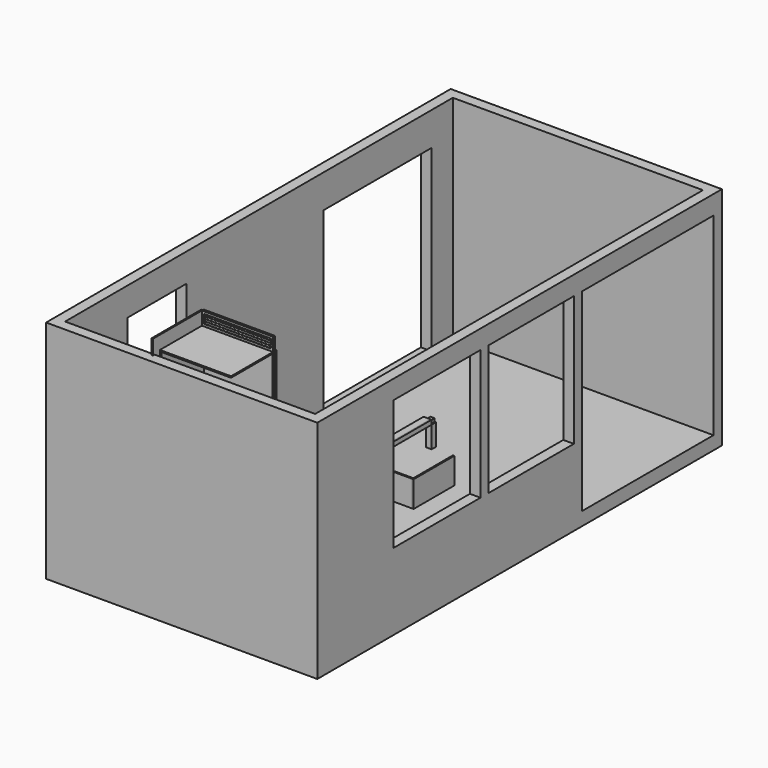
from build123d import *

# Parameters (mm, degrees)
F0_W      = 3098.8
F0_H      = 5778.5
F1_DEPTH  = 152.4
F2_W      = 3098.8
F2_H      = 5778.5
F2_W_2    = 2857.5
F2_H_2    = 5537.2
F3_DEPTH  = 2425.7
F4_W      = 1879.6
F4_H      = 2209.8
F5_DEPTH  = 120.65
F6_W      = 1219.2
F6_H      = 1485.9
F6_W_2    = 1244.6
F7_DEPTH  = 120.65
F8_W      = 844.55
F8_H      = 914.4
F9_DEPTH  = 120.651
F10_W     = 1543.05
F10_H     = 2044.7
F11_DEPTH = 120.651
F13_W     = 812.8
F13_H     = 609.6
F14_DEPTH = 15.875
F15_W     = 781.05
F15_H     = 476.25
F16_DEPTH = 15.875
F15_W_2   = 15.875
F17_DEPTH = 609.6
F18_DEPTH = 15.875
F19_W     = 812.8
F19_H     = 508
F19_W_2   = 781.05
F19_H_2   = 476.25
F19_W_3   = 711.2
F19_H_3   = 406.4
F20_DEPTH = 25.4
F21_W     = 4.7752
F21_H     = 12.7
F24_W     = 736.6
F24_H     = 431.8
F25_DEPTH = 4.7752
F29_W     = 812.8
F29_H     = 152.4
F29_W_2   = 762
F29_H_2   = 101.6
F30_DEPTH = 25.4
F32_DEPTH = 787.4
F34_DEPTH = 15.875
F35_W     = 76.2
F35_H     = 15.875
F36_DEPTH = 984.25
F38_DEPTH = 984.25
F39_W     = 15.875
F39_H     = 50.8
F40_DEPTH = 984.25
F42_DEPTH = 63.5
F43_W     = 565.15
F43_H     = 15.875
F44_DEPTH = 15.875
F45_W     = 609.6
F45_H     = 476.25
F46_DEPTH = 15.875


with BuildPart() as f1:
    # F0 (on Top) → F1 (new body)
    with BuildSketch(Plane.XY):
        Rectangle(F0_W, F0_H)
    extrude(amount=F1_DEPTH)

    # F2 (on face) → F3 (join)
    with BuildSketch(Plane.XY.offset(152.4)):
        Rectangle(F2_W, F2_H)
        Rectangle(F2_W_2, F2_H_2, mode=Mode.SUBTRACT)
    extrude(amount=F3_DEPTH)

    # F4 (on face) → F5 (cut, through all)
    with BuildSketch(Plane.YZ.offset(1549.4)):
        with Locations((1828.8, 1257.3)):
            Rectangle(F4_W, F4_H)
    extrude(amount=-F5_DEPTH, mode=Mode.SUBTRACT)

    # F6 (on face) → F7 (cut, through all)
    with BuildSketch(Plane.YZ.offset(1549.4)):
        with Locations((165.1, 1619.25)):
            Rectangle(F6_W, F6_H)
        with Locations((-1181.1, 1619.25)):
            Rectangle(F6_W_2, F6_H)
    extrude(amount=-F7_DEPTH, mode=Mode.SUBTRACT)

    # F8 (on face) → F9 (cut, through all)
    with BuildSketch(Plane.YZ.offset(-1428.75)):
        with Locations((-1457.325, 1797.05)):
            Rectangle(F8_W, F8_H)
    extrude(amount=-F9_DEPTH, mode=Mode.SUBTRACT)

    # F10 (on face) → F11 (cut, through all)
    with BuildSketch(Plane.YZ.offset(-1428.75)):
        with Locations((1692.275, 1174.75)):
            Rectangle(F10_W, F10_H)
    extrude(amount=-F11_DEPTH, mode=Mode.SUBTRACT)


with BuildPart() as f14:
    # F13 (on face) → F14 (new body)
    with BuildSketch(Plane.XY.offset(2578.1)):
        with Locations((0, -2387.6)):
            Rectangle(F13_W, F13_H)
    extrude(amount=F14_DEPTH)


with BuildPart() as f16:
    # F15 (on face) → F16 (new body)
    with BuildSketch(Plane(origin=(0, -2082.8, 0), x_dir=(-1, 0, 0), z_dir=(0, 1, 0))):
        with Locations((0, 2339.975)):
            Rectangle(F15_W, F15_H)
    extrude(amount=F16_DEPTH)


with BuildPart() as f17:
    # F15 (on face) → F17 (new body, through all)
    with BuildSketch(Plane(origin=(0, -2082.8, 0), x_dir=(-1, 0, 0), z_dir=(0, 1, 0))):
        with Locations((398.4625, 2339.975)):
            Rectangle(F15_W_2, F15_H)
    extrude(amount=-F17_DEPTH)


with BuildPart() as f18:
    # F15 (on face) → F18 (new body)
    with BuildSketch(Plane(origin=(0, -2082.8, 0), x_dir=(-1, 0, 0), z_dir=(0, 1, 0))):
        with Locations((0, 2339.975)):
            Rectangle(F15_W, F15_H)
    extrude(amount=F18_DEPTH)


with BuildPart() as f20:
    # F19 (on face) → F20 (new body)
    with BuildSketch(Plane(origin=(0, -2066.925, 0), x_dir=(-1, 0, 0), z_dir=(0, 1, 0))):
        with Locations((0, 2339.975)):
            Rectangle(F19_W, F19_H)
        with Locations((0, 2339.975)):
            Rectangle(F19_W_2, F19_H_2, mode=Mode.SUBTRACT)
        with Locations((0, 2339.975)):
            Rectangle(F19_W_2, F19_H_2)
        with Locations((0, 2339.975)):
            Rectangle(F19_W_3, F19_H_3, mode=Mode.SUBTRACT)
    extrude(amount=F20_DEPTH)

    # F23: sweep along a path in F22
    with BuildLine(Plane(origin=(0, -2041.525, 0), x_dir=(-1, 0, 0), z_dir=(0, 1, 0))) as f23_path:
        Line((355.6, 2543.175), (-355.6, 2543.175))
        Line((-355.6, 2543.175), (-355.6, 2136.775))
        Line((-355.6, 2136.775), (355.6, 2136.775))
        Line((355.6, 2136.775), (355.6, 2543.175))
    # F21 (on face) → F23 (sweep, cut)
    with BuildSketch(Plane(origin=(355.6, 0, 0), x_dir=(0, -1, 0), z_dir=(-1, 0, 0))):
        with Locations((2043.9126, 2130.425)):
            Rectangle(F21_W, F21_H)
    sweep(path=f23_path.line, transition=Transition.RIGHT, mode=Mode.SUBTRACT)


with BuildPart() as f25:
    # F24 (on face) → F25 (new body)
    with BuildSketch(Plane(origin=(0, -2041.525, 0), x_dir=(-1, 0, 0), z_dir=(0, 1, 0))):
        with Locations((0, 2339.975)):
            Rectangle(F24_W, F24_H)
    extrude(amount=F25_DEPTH)


with BuildPart() as f28:
    # F28: sweep along a path in F26
    with BuildLine(Plane(origin=(0, 0, 2085.975), x_dir=(1, 0, 0), z_dir=(0, 0, -1))) as f28_path:
        Line((63.5, 2066.925), (63.5, 2092.325))
        ThreePointArc((63.5, 2092.325), (59.7802561211, 2101.3052561211), (50.8, 2105.025))
        Line((50.8, 2105.025), (-50.8, 2105.025))
        ThreePointArc((-50.8, 2105.025), (-59.7802561211, 2101.3052561211), (-63.5, 2092.325))
        Line((-63.5, 2092.325), (-63.5, 2066.925))
    # F27 (on face) → F28 (sweep)
    with BuildSketch(Plane.XZ.offset(2066.925)):
        with BuildLine():
            ThreePointArc((57.15, 2085.975), (63.5, 2079.625), (69.85, 2085.975))
            Line((69.85, 2085.975), (57.15, 2085.975))
        make_face()
        with BuildLine():
            Line((57.15, 2085.975), (69.85, 2085.975))
            ThreePointArc((69.85, 2085.975), (63.5, 2092.325), (57.15, 2085.975))
        make_face()
    sweep(path=f28_path.line)


with BuildPart() as f30:
    # F29 (on face) → F30 (new body)
    with BuildSketch(Plane.XZ.offset(2066.925)):
        with Locations((0, 2670.175)):
            Rectangle(F29_W, F29_H)
        with Locations((0, 2670.175)):
            Rectangle(F29_W_2, F29_H_2, mode=Mode.SUBTRACT)
    extrude(amount=F30_DEPTH)

    # F31 (on face) → F32 (join, through all)
    with BuildSketch(Plane(origin=(-406.4, 0, 0), x_dir=(0, -1, 0), z_dir=(-1, 0, 0))):
        with BuildLine():
            Line((2068.3996798487, 2715.0101920908), (2086.3601920908, 2697.0496798487))
            ThreePointArc((2086.3601920908, 2697.0496798487), (2090.8503201513, 2697.0496798487), (2090.8503201513, 2701.5398079092))
            Line((2090.8503201513, 2701.5398079092), (2072.8898079092, 2719.5003201513))
            ThreePointArc((2072.8898079092, 2719.5003201513), (2068.3996798487, 2719.5003201513), (2068.3996798487, 2715.0101920908))
        make_face()
        with BuildLine():
            Line((2068.3996798487, 2689.6101920908), (2086.3601920908, 2671.6496798487))
            ThreePointArc((2086.3601920908, 2671.6496798487), (2090.8503201513, 2671.6496798487), (2090.8503201513, 2676.1398079092))
            Line((2090.8503201513, 2676.1398079092), (2072.8898079092, 2694.1003201513))
            ThreePointArc((2072.8898079092, 2694.1003201513), (2068.3996798487, 2694.1003201513), (2068.3996798487, 2689.6101920908))
        make_face()
        with BuildLine():
            Line((2068.3996798487, 2664.2101920908), (2086.3601920908, 2646.2496798487))
            ThreePointArc((2086.3601920908, 2646.2496798487), (2090.8503201513, 2646.2496798487), (2090.8503201513, 2650.7398079092))
            Line((2090.8503201513, 2650.7398079092), (2072.8898079092, 2668.7003201513))
            ThreePointArc((2072.8898079092, 2668.7003201513), (2068.3996798487, 2668.7003201513), (2068.3996798487, 2664.2101920908))
        make_face()
        with BuildLine():
            Line((2090.8503201513, 2625.3398079092), (2072.8898079092, 2643.3003201513))
            ThreePointArc((2072.8898079092, 2643.3003201513), (2068.3996798487, 2643.3003201513), (2068.3996798487, 2638.8101920908))
            Line((2068.3996798487, 2638.8101920908), (2086.3601920908, 2620.8496798487))
            ThreePointArc((2086.3601920908, 2620.8496798487), (2090.8503201513, 2620.8496798487), (2090.8503201513, 2625.3398079092))
        make_face()
    extrude(amount=-F32_DEPTH)


with BuildPart() as f34:
    # F33 (on Front) → F34 (new body)
    with BuildSketch(Plane.XZ):
        Polygon((335.1245088988, 450.85), (-335.1245088988, 450.85), (-335.1245088988, -450.85), (258.9245088988, -450.85), (258.9245088988, -323.85), (335.1245088988, -323.85), align=None)
    extrude(amount=F34_DEPTH)


with BuildPart() as f36:
    # F35 (on face) → F36 (new body)
    with BuildSketch(Plane(origin=(0, 0, 0), x_dir=(-1, 0, 0), z_dir=(0, 1, 0))):
        with Locations((297.0245088988, 442.9125)):
            Rectangle(F35_W, F35_H)
    extrude(amount=F36_DEPTH)


with BuildPart() as f38:
    # F37 (on face) → F38 (new body)
    with BuildSketch(Plane(origin=(0, 0, 0), x_dir=(-1, 0, 0), z_dir=(0, 1, 0))):
        Polygon((335.1245088988, -307.975), (-335.1245088988, -307.975), (-335.1245088988, -323.85), (-258.9245088988, -323.85), (335.1245088988, -323.85), align=None)
    extrude(amount=F38_DEPTH)


with BuildPart() as f40:
    # F39 (on face) → F40 (new body)
    with BuildSketch(Plane(origin=(0, 0, 0), x_dir=(-1, 0, 0), z_dir=(0, 1, 0))):
        with Locations((250.9870088988, 425.45)):
            Rectangle(F39_W, F39_H)
    extrude(amount=F40_DEPTH)


with BuildPart() as f42:
    # F41 (on face) → F42 (new body)
    with BuildSketch(Plane(origin=(0, 984.25, 0), x_dir=(-1, 0, 0), z_dir=(0, 1, 0))):
        Polygon((243.0495088988, 400.05), (243.0495088988, -307.975), (306.5495088988, -307.975), (306.5495088988, 434.975), (258.9245088988, 434.975), (258.9245088988, 400.05), align=None)
    extrude(amount=F42_DEPTH)


with BuildPart() as f44:
    # F43 (on face) → F44 (new body)
    with BuildSketch(Plane.YZ.offset(335.1245088988)):
        Polygon((565.15, 450.85), (-15.875, 450.85), (-15.875, -323.85), (0, -323.85), (0, -307.975), (565.15, -307.975), align=None)
        with Locations((282.575, -315.9125)):
            Rectangle(F43_W, F43_H)
    extrude(amount=F44_DEPTH)


with BuildPart() as f46:
    # F45 (on face) → F46 (new body)
    with BuildSketch(Plane(origin=(-406.4, 0, 0), x_dir=(0, -1, 0), z_dir=(-1, 0, 0))):
        Polygon((2794, 2746.375), (2082.8, 2746.375), (2082.8, 2578.1), (2692.4, 2578.1), (2692.4, 2101.85), (2082.8, 2101.85), (2082.8, 346.075), (2794, 346.075), align=None)
        with Locations((2387.6, 2339.975)):
            Rectangle(F45_W, F45_H)
    extrude(amount=F46_DEPTH)


solid = Compound([f1.part, f14.part, f16.part, f17.part, f18.part, f20.part, f25.part, f28.part, f30.part, f34.part, f36.part, f38.part, f40.part, f42.part, f44.part, f46.part])
